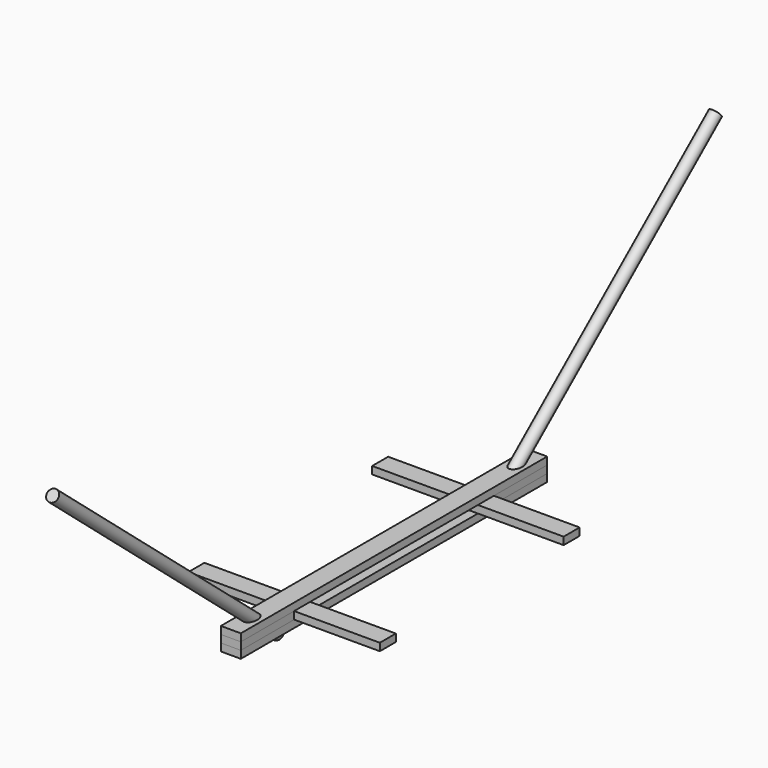
from build123d import *

# Parameters (mm, degrees)
F1_DEPTH = 120
F2_DEPTH = 120
F3_DEPTH = 120
F0_W     = 120
F0_H     = 45
F4_DEPTH = 1150


# Not quite as in the source:
# - ends of sketch curves that miss each other by under 0.0002 mm in the source are joined


with BuildPart() as f1:
    # F0 (on Right) → F1 (new body)
    with BuildSketch(Plane.YZ):
        Polygon((1919.027900419, 135), (1819.027900419, 135), (1765.3989887522, 90), (1919.027900419, 90), align=None)
        Polygon((-227.3431879143, 90), (-172.8928539742, 90), (-226.5217656409, 135), (-280.972099581, 135), align=None)
        Polygon((1764.5775664789, 135), (1710.1272325387, 135), (1656.498320872, 90), (1710.9486548121, 90), align=None)
        Polygon((-380.972099581, 90), (-227.3431879143, 90), (-280.972099581, 135), (-380.972099581, 135), align=None)
        Polygon((-118.4425200341, 90), (19.027900419, 90), (139.027900419, 90), (1399.027900419, 90), (1519.027900419, 90), (1656.498320872, 90), (1710.1272325387, 135), (-172.0714317008, 135), align=None)
        Polygon((-172.8928539742, 90), (-118.4425200341, 90), (-172.0714317008, 135), (-226.5217656409, 135), align=None)
        Polygon((1819.027900419, 135), (1764.5775664789, 135), (1710.9486548121, 90), (1765.3989887522, 90), align=None)
    extrude(amount=F1_DEPTH)


with BuildPart() as f2:
    # F0 (on Right) → F2 (new body)
    with BuildSketch(Plane.YZ):
        Polygon((-120.0853645808, 0), (-173.7142762475, 45), (-380.972099581, 45), (-380.972099581, 0), align=None)
        Polygon((-65.6350306407, 0), (-119.2639423074, 45), (-173.7142762475, 45), (-120.0853645808, 0), align=None)
        Polygon((1711.7700770855, 45), (1658.1411654188, 0), (1919.027900419, 0), (1919.027900419, 45), align=None)
        Polygon((139.027900419, 45), (19.027900419, 45), (-64.8136083673, 45), (-11.1847011409, 3.7259e-06), (1549.2405019789, 0), (1602.8694092053, 45), (1519.027900419, 45), (1399.027900419, 45), align=None)
        Polygon((1602.8694092053, 45), (1549.2405019789, 3.7259e-06), (1603.6908314786, 0), (1657.3197431454, 45), align=None)
        Polygon((1657.3197431454, 45), (1603.6908314786, 0), (1658.1411654188, 0), (1711.7700770855, 45), align=None)
        Polygon((-11.1847011409, 3.7259e-06), (-64.8136083673, 45), (-119.2639423074, 45), (-65.6350306407, 0), align=None)
    extrude(amount=F2_DEPTH)


with BuildPart() as f3:
    # F0 (on Right) → F3 (new body)
    with BuildSketch(Plane.YZ):
        Polygon((-380.972099581, 45), (-173.7142762475, 45), (-227.3431879143, 90), (-380.972099581, 90), align=None)
        Polygon((-173.7142762475, 45), (-119.2639423074, 45), (-172.8928539742, 90), (-227.3431879143, 90), align=None)
        Polygon((-119.2639423074, 45), (-64.8136083673, 45), (-118.4425200341, 90), (-172.8928539742, 90), align=None)
        Polygon((-64.8136083673, 45), (19.027900419, 45), (19.027900419, 90), (-118.4425200341, 90), align=None)
    extrude(amount=F3_DEPTH)


with BuildPart() as f3b:
    # F0 (on Right) → F3, piece 2 (new body)
    with BuildSketch(Plane.YZ):
        Polygon((1519.027900419, 90), (1519.027900419, 45), (1602.8694092053, 45), (1656.498320872, 90), align=None)
        Polygon((1656.498320872, 90), (1602.8694092053, 45), (1657.3197431454, 45), (1710.9486548121, 90), align=None)
        Polygon((1710.9486548121, 90), (1657.3197431454, 45), (1711.7700770855, 45), (1765.3989887522, 90), align=None)
        Polygon((1765.3989887522, 90), (1711.7700770855, 45), (1919.027900419, 45), (1919.027900419, 90), align=None)
    extrude(amount=F3_DEPTH)


with BuildPart() as f4:
    # F0 (on Right) → F4 (new body)
    with BuildSketch(Plane.YZ):
        with Locations((79.027900419, 67.5)):
            Rectangle(F0_W, F0_H)
    extrude(amount=F4_DEPTH)


with BuildPart() as f4b:
    # F0 (on Right) → F4, piece 2 (new body)
    with BuildSketch(Plane.YZ):
        with Locations((1459.027900419, 67.5)):
            Rectangle(F0_W, F0_H)
    extrude(amount=F4_DEPTH)


with BuildPart() as f4b_1:
    # F5: moved
    add(f4b.part.moved(Location((-515, 0, 0))))


with BuildPart() as f4_1:
    # F5: moved
    add(f4.part.moved(Location((-515, 0, 0))))


with BuildPart() as f6:
    # F0 (on Right) → F6 (revolve)
    with BuildSketch(Plane.YZ):
        Polygon((-227.3431879143, 90), (-172.8928539742, 90), (-226.5217656409, 135), (-280.972099581, 135), align=None)
        Polygon((-173.7142762475, 45), (-119.2639423074, 45), (-172.8928539742, 90), (-227.3431879143, 90), align=None)
        Polygon((-65.6350306407, 0), (-119.2639423074, 45), (-173.7142762475, 45), (-120.0853645808, 0), align=None)
        Polygon((-33.6822674799, -26.8115517833), (-65.6350306407, 0), (-120.0853645808, 0), (-56.179833819, -53.6231072924), align=None)
        Polygon((-280.972099581, 135), (-226.5217656409, 135), (-1718.9800423417, 1387.3211895271), (-1741.4776086807, 1360.5096340179), align=None)
    revolve(axis=Axis((0, -876.3311549108, 680.2548188719), (0, 0.7660444431, -0.6427876097)))


with BuildPart() as f7:
    # F0 (on Right) → F7 (revolve)
    with BuildSketch(Plane.YZ):
        Polygon((1658.1411654188, 0), (1603.6908314786, 0), (1571.7380683179, -26.8115517833), (1594.2356346569, -53.6231072924), align=None)
        Polygon((1657.3197431454, 45), (1603.6908314786, 0), (1658.1411654188, 0), (1711.7700770855, 45), align=None)
        Polygon((1710.9486548121, 90), (1657.3197431454, 45), (1711.7700770855, 45), (1765.3989887522, 90), align=None)
        Polygon((1819.027900419, 135), (1764.5775664789, 135), (1710.9486548121, 90), (1765.3989887522, 90), align=None)
        Polygon((3257.0358431796, 1387.3211895271), (1764.5775664789, 135), (1819.027900419, 135), (3279.5334095187, 1360.5096340179), align=None)
    revolve(axis=Axis((0, 2414.3869557488, 680.2548188719), (0, -0.7660444431, -0.6427876097)))


with BuildPart() as f6_1:
    # F8: moved
    add(f6.part.moved(Location((60, 0, 0))))


with BuildPart() as f7_1:
    # F8: moved
    add(f7.part.moved(Location((60, 0, 0))))


solid = Compound([f1.part, f2.part, f3.part, f3b.part, f4b_1.part, f4_1.part, f6_1.part, f7_1.part])
